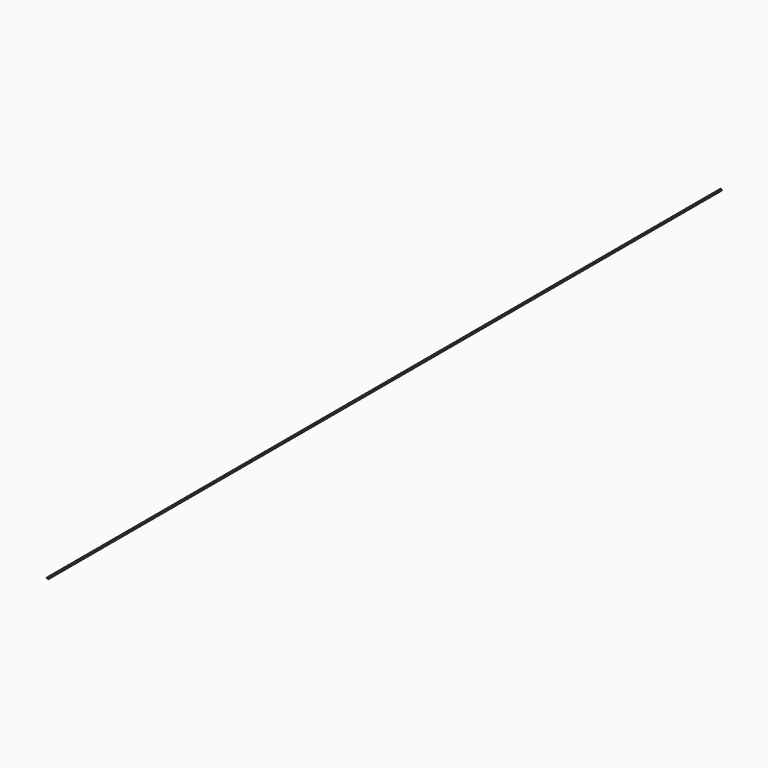
from build123d import *

# Parameters (mm, degrees)
F1_DEPTH = 254
F3_DEPTH = 98.298
F4_R     = 45.7936330536
F5_DEPTH = 254000
F4_W     = 34.1130308807
F4_H     = 52.4815917015
F4_W_2   = 31.4889550209
F4_R_2   = 48.4078793894


with BuildPart() as f1:
    # F0 (on Front) → F1 (new body)
    with BuildSketch(Plane.XZ):
        with BuildLine():
            add(Edge.make_bspline(
                [(-132.4997842312, -33.1585071981), (-94.8715670758, -55.7691471996), (75.2931336197, 11.6570935994), (-158.0532035393, 118.3232014636), (-164.9381428441, -13.6664317217), (-132.4997842312, -33.1585071981)],
                knots=[0, 0, 0, 0, 0.3508604639, 0.6975318415, 1, 1, 1, 1], degree=3))
        make_face()
    extrude(amount=F1_DEPTH)

    # F2 (on Front) → F3 (join)
    with BuildSketch(Plane.XZ):
        Polygon((18.7816545367, 236.3309338689), (0, 295.0955033302), (0, 236.3309338689), align=None)
        Polygon((-43.7029358283, 208.7382471013), (0, 295.0955033302), (-133.6115300655, 155.4528772831), (-131.6725555099, 153.1969404377), (-128.0994687707, 155.4528772831), align=None)
        Polygon((0, 236.3309338689), (0, 295.0955033302), (-43.7029358283, 208.7382471013), align=None)
        Polygon((16.7047991803, 210.1977108919), (18.7816545367, 236.3309338689), (0, 236.3309338689), align=None)
        Polygon((37.5633090734, 177.5663644075), (18.7816545367, 236.3309338689), (16.7047991803, 210.1977108919), align=None)
        Polygon((0, 0), (37.5633090734, 177.5663644075), (13.8400442615, 174.1502900454), align=None)
        Polygon((13.8400442615, 174.1502900454), (37.5633090734, 177.5663644075), (16.7047991803, 210.1977108919), align=None)
        Polygon((13.8400442615, 174.1502900454), (0, 172.1573678761), (0, 0), align=None)
        Polygon((0, 0), (0, 172.1573678761), (-67.1056383852, 162.4943702804), (-2.81803512, 129.9602541824), (-2.81803512, 126.7872303724), (-9.087948685, 129.9602541824), (-47.6953043341, 117.6210160492), (-57.8791172117, 141.1642400595), (-123.0878839493, 154.4331057234), (-131.6725555099, 153.1969404377), align=None)
        Polygon((-128.0994687707, 155.4528772831), (-131.6725555099, 153.1969404377), (-123.0878839493, 154.4331057234), align=None)
    extrude(amount=F3_DEPTH)

    # F4 (on Front) → F5, piece 6 (join)
    with BuildSketch(Plane.XZ):
        with Locations((-141.1879509687, 129.2051970959)):
            Circle(F4_R_2)
    extrude(amount=F5_DEPTH)


with BuildPart() as f5:
    # F4 (on Front) → F5 (new body)
    with BuildSketch(Plane.XZ):
        with Locations((108.2467138767, 65.2941092849)):
            Circle(F4_R)
    extrude(amount=F5_DEPTH)


with BuildPart() as f5b:
    # F4 (on Front) → F5, piece 2 (new body)
    with BuildSketch(Plane.XZ):
        Polygon((86.0063657165, -74.0351453424), (86.0063657165, -26.9379392266), (55.9164769948, -26.9379392266), (55.9164769948, -41.9828779995), (55.9164769948, -75.3434002399), align=None)
    extrude(amount=F5_DEPTH)


with BuildPart() as f5c:
    # F4 (on Front) → F5, piece 3 (new body)
    with BuildSketch(Plane.XZ):
        with Locations((-71.6498289257, 399.4854092598)):
            Rectangle(F4_W, F4_H)
    extrude(amount=F5_DEPTH)


with BuildPart() as f5d:
    # F4 (on Front) → F5, piece 4 (new body)
    with BuildSketch(Plane.XZ):
        with Locations((-116.2591874599, 399.4854092598)):
            Rectangle(F4_W_2, F4_H)
    extrude(amount=F5_DEPTH)


with BuildPart() as f5e:
    # F4 (on Front) → F5, piece 5 (new body)
    with BuildSketch(Plane.XZ):
        with BuildLine():
            ThreePointArc((-106.5903799208, 277.4657011032), (-93.9545035362, 274.0478505444), (-81.3186271516, 277.4657011032))
            Line((-81.3186271516, 277.4657011032), (-106.5903799208, 277.4657011032))
        make_face()
        with BuildLine():
            Line((-106.5903799208, 277.4657011032), (-81.3186271516, 277.4657011032))
            ThreePointArc((-81.3186271516, 277.4657011032), (-72.2166751713, 286.6325182054), (-68.8880075764, 299.1143465042))
            ThreePointArc((-68.8880075764, 299.1143465042), (-106.436331835, 320.8521748692), (-106.5903799208, 277.4657011032))
        make_face()
    extrude(amount=F5_DEPTH)


with BuildPart() as f5f:
    # F4 (on Front) → F5, piece 7 (new body)
    with BuildSketch(Plane.XZ):
        Polygon((-290.8359467983, 240.2228713036), (-416.4027481818, 184.9071007683), (-414.843598616, 166.6558539839), (-353.4996639846, 179.548478343), align=None)
        Polygon((-414.843598616, 166.6558539839), (-416.4027481818, 184.9071007683), (-497.05478549, 149.3775695562), align=None)
    extrude(amount=F5_DEPTH)


solid = Compound([f1.part, f5.part, f5b.part, f5c.part, f5d.part, f5e.part, f5f.part])
